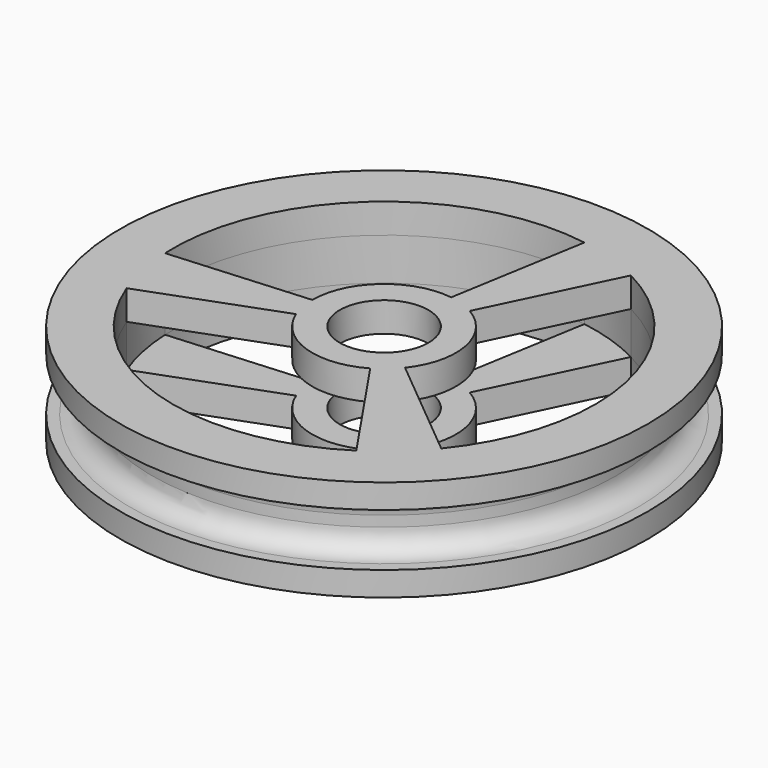
from build123d import *
from build123d import SkipClean  # not in build123d's __all__

# Parameters (mm, degrees)
F0_R     = 15.875
F1_DEPTH = 3.048
F2_R     = 17.9958283003
F2_R_2   = 13.97
F3_DEPTH = 1.5875
F4_R     = 2.667
F5_DEPTH = 6.097
F6_R     = 1.27
F7_R     = 12.7
F8_DEPTH = 1.27


with BuildPart() as f1:
    # F0 (on Top) → F1 (new body, symmetric)
    with BuildSketch(Plane.XY):
        Circle(F0_R)
    extrude(amount=F1_DEPTH, both=True)

    # F2 (on Top) → F3 (cut, symmetric)
    with BuildSketch(Plane.XY):
        Circle(F2_R)
        Circle(F2_R_2, mode=Mode.SUBTRACT)
    extrude(amount=F3_DEPTH, both=True, mode=Mode.SUBTRACT)

    # F4 (on face) → F5 (cut, through all)
    with BuildSketch(Plane.XY.offset(3.048)):
        with BuildLine():
            Line((0.6120390991, 4.2744043025), (2.0170417977, 12.5388014733))
            ThreePointArc((2.0170417977, 12.5388014733), (-8.4665969818, 9.4660834323), (-12.6852858441, -0.6111653244))
            Line((-12.6852858441, -0.6111653244), (-4.318, 0))
            ThreePointArc((-4.318, 0), (-2.8286338726, 3.2625073816), (0.6120390991, 4.2744043025))
        make_face()
        Circle(F4_R)
        with BuildLine():
            ThreePointArc((2.159, -3.7394976935), (-1.4110973362, -4.0809224824), (-4.0077622616, -1.6071607433))
            Line((-4.0077622616, -1.6071607433), (-11.8674415077, -4.5225912993))
            ThreePointArc((-11.8674415077, -4.5225912993), (-3.9645702358, -12.065329786), (6.8719276189, -10.6801971331))
            Line((6.8719276189, -10.6801971331), (2.159, -3.7394976935))
        make_face()
        with BuildLine():
            ThreePointArc((2.159, 3.7394976935), (4.2397312088, 0.8184151008), (3.3957231624, -2.6672435592))
            Line((3.3957231624, -2.6672435592), (9.85039971, -8.016210174))
            ThreePointArc((9.85039971, -8.016210174), (12.4311672176, 2.5992463537), (5.8133582252, 11.2913624574))
            Line((5.8133582252, 11.2913624574), (2.159, 3.7394976935))
        make_face()
    extrude(amount=-F5_DEPTH, mode=Mode.SUBTRACT)

    # F6
    f6_edges = [f1.edges().sort_by_distance(p)[0] for p in [
        (-13.97, 0, -1.5875),
        (-13.97, 0, 1.5875),
    ]]
    fillet(f6_edges, radius=F6_R)

    # F7 (on Top) → F8 (cut, symmetric)
    with BuildSketch(Plane.XY):
        Circle(F7_R)
    with SkipClean():  # cleaning this boolean's faces spoils the solid; the shape is the same uncleaned
        extrude(amount=F8_DEPTH, both=True, mode=Mode.SUBTRACT)


solid = f1.part
